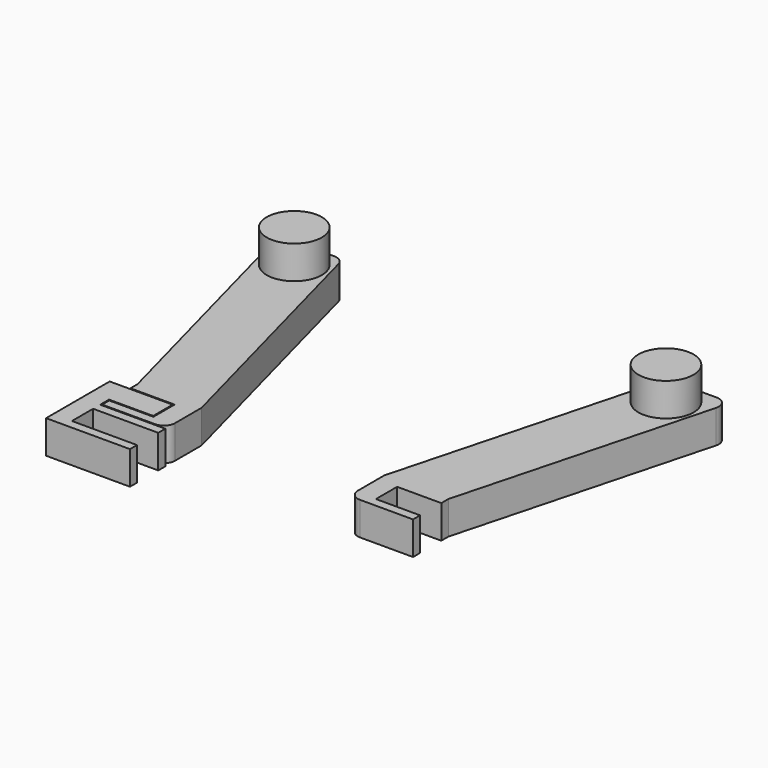
from build123d import *

# Parameters (mm, degrees)
F0_R     = 12.5
F1_DEPTH = 15
F2_DEPTH = 30
F3_R     = 5
F0_W     = 29.5
F0_H     = 4
F5_DEPTH = 15


# Not quite as in the source:
# - a feature names something its author has since deleted; it is built from what else it names


with BuildPart() as f1:
    # F0 (on Top) → F1 (new body)
    with BuildSketch(Plane.XY):
        Polygon((-70.3989224725, -16), (-70.3989224725, -20), (-41.3989224725, -20), (-41.3989224725, 0), (-70.3989224725, 0), (-70.3989224725, -4), (-50.3989224725, -4), (-50.3989224725, -16), align=None)
        Polygon((-70.3989224725, 0), (-41.3989224725, 0), (-73.4119985036, 120), (-102.4119985036, 120), align=None)
        with Locations((-84.1744648133, 105.989973522)):
            Circle(F0_R, mode=Mode.SUBTRACT)
    extrude(amount=F1_DEPTH)

    # F0 (on Top) → F2 (join)
    with BuildSketch(Plane.XY):
        with Locations((-84.1744648133, 105.989973522)):
            Circle(F0_R)
    extrude(amount=F2_DEPTH)

    # F3
    f3_edges = [f1.edges().sort_by_distance(p)[0] for p in [
        (-41.398922, -20, 7.5),
        (-73.411999, 120, 7.5),
        (-102.411999, 120, 7.5),
    ]]
    fillet(f3_edges, radius=F3_R)


with BuildPart() as f4_1:
    # F4: instance of F1
    add(f1.part.mirror(Plane.YZ))


with BuildPart() as f5:
    # F0 (on Top) → F5 (new body)
    with BuildSketch(Plane.XY):
        Polygon((-70.8989224725, -15.5), (-79.3989224725, -15.5), (-79.3989224725, -40.5), (-41.3989224725, -40.5), (-41.3989224725, -36.5), (-70.8989224725, -36.5), (-70.8989224725, -24.5), (-70.8989224725, -20.5), align=None)
        Polygon((-50.8989224725, -15.5), (-50.8989224725, -4.5), (-79.3989224725, -4.5), (-79.3989224725, -15.5), (-70.8989224725, -15.5), align=None)
        with Locations((-56.1489224725, -22.5)):
            Rectangle(F0_W, F0_H)
    extrude(amount=F5_DEPTH)


solid = Compound([f1.part, f4_1.part, f5.part])
